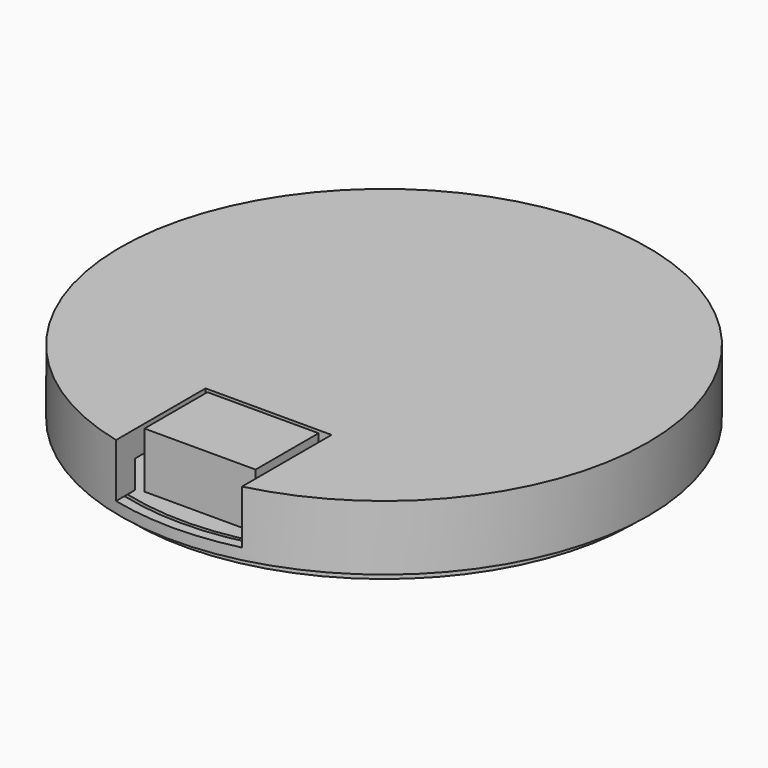
from build123d import *

# Parameters (mm, degrees)
F0_R     = 13.5
F0_W     = 6
F0_H     = 4.25
F1_DEPTH = 1.2
F2_DEPTH = 4.2
F3_R     = 14.25
F3_R_2   = 13.7
F3_R_3   = 13.5
F4_DEPTH = 2.9
F5_DEPTH = 0.6
F3_W     = 6
F3_H     = 4.25
F6_DEPTH = 1.5
F7_W     = 6.8
F7_H     = 3
F8_DEPTH = 8


with BuildPart() as f1:
    # F0 (on Top) → F1 (new body)
    with BuildSketch(Plane.XY):
        Circle(F0_R)
        with Locations((0, -10.295)):
            Rectangle(F0_W, F0_H, mode=Mode.SUBTRACT)
        with Locations((0, -10.295)):
            Rectangle(F0_W, F0_H)
    extrude(amount=F1_DEPTH)

    # F0 (on Top) → F2 (join)
    with BuildSketch(Plane.XY):
        with Locations((0, -10.295)):
            Rectangle(F0_W, F0_H)
    extrude(amount=F2_DEPTH)


with BuildPart() as f4:
    # F3 (on face) → F4 (new body)
    with BuildSketch(Plane.XY.offset(1.2)):
        Circle(F3_R)
        Circle(F3_R_2, mode=Mode.SUBTRACT)
        Circle(F3_R_2)
        Circle(F3_R_3, mode=Mode.SUBTRACT)
        Circle(F3_R_3)
        with BuildLine():
            Line((3.4, -12.5475097131), (3.4, -12.795))
            Line((3.4, -12.795), (2.2995597405, -12.795))
            ThreePointArc((2.2995597405, -12.795), (0, -13), (-2.2995597405, -12.795))
            Line((-2.2995597405, -12.795), (-3.4, -12.795))
            Line((-3.4, -12.795), (-3.4, -12.5475097131))
            ThreePointArc((-3.4, -12.5475097131), (-7.8993670633, 10.3247275993), (13, 0))
            ThreePointArc((13, 0), (10.3247275993, -7.8993670633), (3.4, -12.5475097131))
        make_face(mode=Mode.SUBTRACT)
        with BuildLine():
            Line((3.4, -7.795), (3.4, -12.5475097131))
            ThreePointArc((3.4, -12.5475097131), (10.3247275993, -7.8993670633), (13, 0))
            ThreePointArc((13, 0), (-7.8993670633, 10.3247275993), (-3.4, -12.5475097131))
            Line((-3.4, -12.5475097131), (-3.4, -7.795))
            Line((-3.4, -7.795), (3.4, -7.795))
        make_face()
        with BuildLine():
            ThreePointArc((-2.2995597405, -12.795), (0, -13), (2.2995597405, -12.795))
            Line((2.2995597405, -12.795), (-2.2995597405, -12.795))
        make_face()
    extrude(amount=F4_DEPTH)

    # F3 (on face) → F5 (join)
    with BuildSketch(Plane.XY.offset(1.2)):
        Circle(F3_R)
        Circle(F3_R_2, mode=Mode.SUBTRACT)
    extrude(amount=-F5_DEPTH)

    # F3 (on face) → F6 (cut)
    with BuildSketch(Plane.XY.offset(1.2)):
        with BuildLine():
            Line((3.4, -7.795), (3.4, -12.5475097131))
            ThreePointArc((3.4, -12.5475097131), (10.3247275993, -7.8993670633), (13, 0))
            ThreePointArc((13, 0), (-7.8993670633, 10.3247275993), (-3.4, -12.5475097131))
            Line((-3.4, -12.5475097131), (-3.4, -7.795))
            Line((-3.4, -7.795), (3.4, -7.795))
        make_face()
        with BuildLine():
            Line((-2.2995597405, -12.795), (2.2995597405, -12.795))
            ThreePointArc((2.2995597405, -12.795), (2.8524652793, -12.6831952532), (3.4, -12.5475097131))
            Line((3.4, -12.5475097131), (3.4, -7.795))
            Line((3.4, -7.795), (-3.4, -7.795))
            Line((-3.4, -7.795), (-3.4, -12.5475097131))
            ThreePointArc((-3.4, -12.5475097131), (-2.8524652793, -12.6831952532), (-2.2995597405, -12.795))
        make_face()
        with Locations((0, -10.295)):
            Rectangle(F3_W, F3_H, mode=Mode.SUBTRACT)
        with BuildLine():
            ThreePointArc((-2.2995597405, -12.795), (0, -13), (2.2995597405, -12.795))
            Line((2.2995597405, -12.795), (-2.2995597405, -12.795))
        make_face()
    extrude(amount=F6_DEPTH, mode=Mode.SUBTRACT)

    # F7 (on face) → F8 (cut)
    with BuildSketch(Plane.XZ.offset(12.42)):
        with Locations((0, 2.7)):
            Rectangle(F7_W, F7_H)
    extrude(amount=F8_DEPTH, mode=Mode.SUBTRACT)


solid = Compound([f1.part, f4.part])
